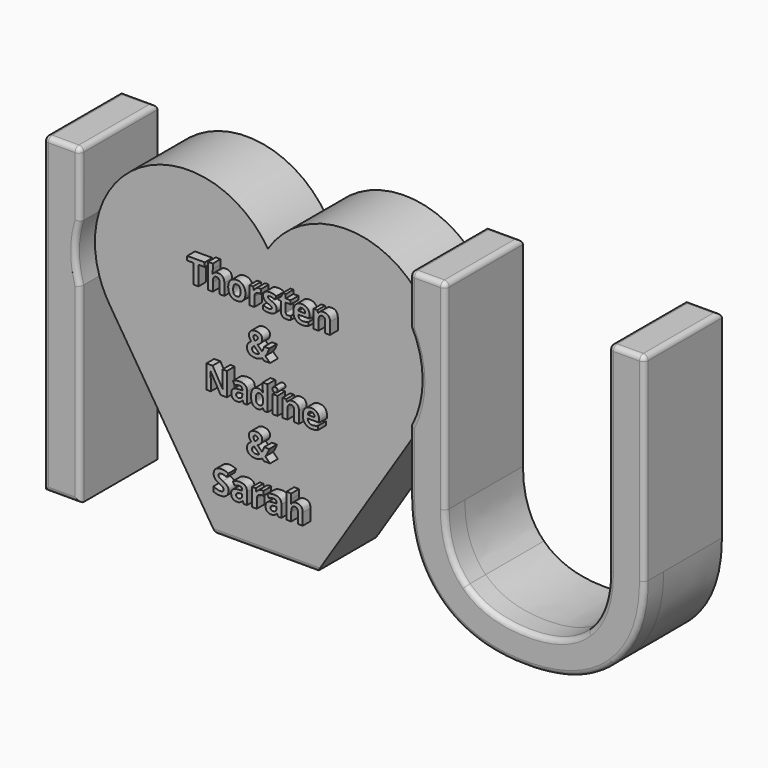
from build123d import *

# Parameters (mm, degrees)
F1_DEPTH     = 15
F2_TEXT_SIZE = 6.6989986393
F3_DEPTH     = 17
F4_R         = 1
F5_DEPTH     = 20
F6_R         = 1


# Not quite as in the source:
# - a feature names something its author has since deleted; it is built from what else it names
# - Text() gives the source's letters only with a copy of the font that has no kerning and outlines rounded to 1/6400 em; it was checked with that copy


with BuildPart() as f1:
    # F0 (on Front) → F1 (new body)
    with BuildSketch(Plane.XZ):
        with BuildLine():
            Line((-32.6601865779, 34.9033940146), (-10.6569835838, 0.1944517979))
            Line((-10.6569835838, 0.1944517979), (10.1186365179, 0.1944517979))
            Line((10.1186365179, 0.1944517979), (32.3398134221, 34.9033940146))
            ThreePointArc((32.3398134221, 34.9033940146), (32.7910788138, 35.6446323114), (33.2083891795, 36.4055046561))
            Line((33.2083891795, 36.4055046561), (33.2083891795, 54.1057090688))
            ThreePointArc((33.2083891795, 54.1057090688), (17.0374838295, 64.4358441872), (0, 55.6078197103))
            ThreePointArc((0, 55.6078197103), (-18.8035868283, 64.4316879893), (-34.7526041667, 51.1251341547))
            Line((-34.7526041667, 51.1251341547), (-34.7526041667, 39.3860795702))
            ThreePointArc((-34.7526041667, 39.3860795702), (-33.8503527488, 37.0775407014), (-32.6601865779, 34.9033940146))
        make_face()
        with BuildLine():
            Line((-34.7526041667, 0), (-34.7526041667, 39.3860795702))
            ThreePointArc((-34.7526041667, 39.3860795702), (-35.6650424142, 45.2556068624), (-34.7526041667, 51.1251341547))
            Line((-34.7526041667, 51.1251341547), (-34.7526041667, 64.4498697917))
            Line((-34.7526041667, 64.4498697917), (-42.2428385417, 64.4498697917))
            Line((-42.2428385417, 64.4498697917), (-42.2428385417, 0))
            Line((-42.2428385417, 0), (-34.7526041667, 0))
        make_face()
        with BuildLine():
            ThreePointArc((-34.7526041667, 51.1251341547), (-35.6650424142, 45.2556068624), (-34.7526041667, 39.3860795702))
            Line((-34.7526041667, 39.3860795702), (-34.7526041667, 51.1251341547))
        make_face()
        with BuildLine():
            Line((33.2083891795, 54.1057090688), (33.2083891795, 36.4055046561))
            ThreePointArc((33.2083891795, 36.4055046561), (35.3697555097, 45.2556068624), (33.2083891795, 54.1057090688))
        make_face()
        with BuildLine():
            ThreePointArc((33.2083891795, 54.1057090688), (35.3697555097, 45.2556068624), (33.2083891795, 36.4055046561))
            Line((33.2083891795, 36.4055046561), (33.2083891795, 23.742953204))
            add(Edge.make_bspline(
                [(39.4529606271, 6.6274334554), (33.2083891795, 12.8581741801), (33.2083891795, 23.742953204)],
                knots=[0, 0, 0, 1, 1, 1], degree=2))
            add(Edge.make_bspline(
                [(57.1078785739, 0.3966927308), (45.6975320748, 0.3966927308), (39.4529606271, 6.6274334554)],
                knots=[0, 0, 0, 1, 1, 1], degree=2))
            add(Edge.make_bspline(
                [(75.0463263427, 6.5790259248), (68.5182250729, 0.3966927308), (57.1078785739, 0.3966927308)],
                knots=[0, 0, 0, 1, 1, 1], degree=2))
            add(Edge.make_bspline(
                [(81.5744276124, 23.5769845277), (81.5744276124, 12.7613591189), (75.0463263427, 6.5790259248)],
                knots=[0, 0, 0, 1, 1, 1], degree=2))
            Line((81.5744276124, 23.5769845277), (81.5744276124, 64.4606018019))
            Line((81.5744276124, 64.4606018019), (74.230313684, 64.4606018019))
            Line((74.230313684, 64.4606018019), (74.230313684, 23.3142007901))
            add(Edge.make_bspline(
                [(69.9082127373, 11.1016723554), (74.230313684, 15.3615350483), (74.230313684, 23.3142007901)],
                knots=[0, 0, 0, 1, 1, 1], degree=2))
            add(Edge.make_bspline(
                [(57.5919538799, 6.8418096624), (65.5861117907, 6.8418096624), (69.9082127373, 11.1016723554)],
                knots=[0, 0, 0, 1, 1, 1], degree=2))
            add(Edge.make_bspline(
                [(44.8884347776, 11.0809262708), (49.2105357242, 6.8418096624), (57.5919538799, 6.8418096624)],
                knots=[0, 0, 0, 1, 1, 1], degree=2))
            add(Edge.make_bspline(
                [(40.566333831, 23.2312164519), (40.566333831, 15.3200428793), (44.8884347776, 11.0809262708)],
                knots=[0, 0, 0, 1, 1, 1], degree=2))
            Line((40.566333831, 23.2312164519), (40.566333831, 64.4606018019))
            Line((40.566333831, 64.4606018019), (33.2083891795, 64.4606018019))
            Line((33.2083891795, 64.4606018019), (33.2083891795, 54.1057090688))
        make_face()
    extrude(amount=F1_DEPTH)

    # F2 (on Front) → F3 (join)
    with BuildSketch(Plane.XZ):
        with Locations((-15.1669165656, 45.46367671)):
            Text('Thorsten', F2_TEXT_SIZE, font='Open Sans', font_style=FontStyle.BOLD, text_align=(TextAlign.LEFT, TextAlign.BOTTOM))
        with Locations((-2.9820660719, 36.3530385606)):
            Text('&', F2_TEXT_SIZE, font='Open Sans', font_style=FontStyle.BOLD, text_align=(TextAlign.LEFT, TextAlign.BOTTOM))
        with Locations((-11.6855307103, 27.2424004112)):
            Text('Nadine', F2_TEXT_SIZE, font='Open Sans', font_style=FontStyle.BOLD, text_align=(TextAlign.LEFT, TextAlign.BOTTOM))
        with Locations((-2.9820660719, 18.1317622618)):
            Text('&', F2_TEXT_SIZE, font='Open Sans', font_style=FontStyle.BOLD, text_align=(TextAlign.LEFT, TextAlign.BOTTOM))
        with Locations((-9.9448377826, 9.0211241124)):
            Text('Sarah', F2_TEXT_SIZE, font='Open Sans', font_style=FontStyle.BOLD, text_align=(TextAlign.LEFT, TextAlign.BOTTOM))
    extrude(amount=F3_DEPTH)

    # F4
    f4_edges = [f1.edges().sort_by_distance(p)[0] for p in [
        (-34.752604, -7.5, 64.44987),
        (-42.242839, -7.5, 64.44987),
        (-42.242839, -7.5, 0),
        (-34.752604, -7.5, 0),
        (-38.497721, 0, 64.44987),
        (-38.497721, 0, 0),
    ]]
    fillet(f4_edges, radius=F4_R)

    # F0 (on Front) → F5 (join)
    with BuildSketch(Plane.XZ):
        with BuildLine():
            Line((-34.7526041667, 0), (-34.7526041667, 39.3860795702))
            ThreePointArc((-34.7526041667, 39.3860795702), (-35.6650424142, 45.2556068624), (-34.7526041667, 51.1251341547))
            Line((-34.7526041667, 51.1251341547), (-34.7526041667, 64.4498697917))
            Line((-34.7526041667, 64.4498697917), (-42.2428385417, 64.4498697917))
            Line((-42.2428385417, 64.4498697917), (-42.2428385417, 0))
            Line((-42.2428385417, 0), (-34.7526041667, 0))
        make_face()
        with BuildLine():
            ThreePointArc((33.2083891795, 54.1057090688), (35.3697555097, 45.2556068624), (33.2083891795, 36.4055046561))
            Line((33.2083891795, 36.4055046561), (33.2083891795, 23.742953204))
            add(Edge.make_bspline(
                [(39.4529606271, 6.6274334554), (33.2083891795, 12.8581741801), (33.2083891795, 23.742953204)],
                knots=[0, 0, 0, 1, 1, 1], degree=2))
            add(Edge.make_bspline(
                [(57.1078785739, 0.3966927308), (45.6975320748, 0.3966927308), (39.4529606271, 6.6274334554)],
                knots=[0, 0, 0, 1, 1, 1], degree=2))
            add(Edge.make_bspline(
                [(75.0463263427, 6.5790259248), (68.5182250729, 0.3966927308), (57.1078785739, 0.3966927308)],
                knots=[0, 0, 0, 1, 1, 1], degree=2))
            add(Edge.make_bspline(
                [(81.5744276124, 23.5769845277), (81.5744276124, 12.7613591189), (75.0463263427, 6.5790259248)],
                knots=[0, 0, 0, 1, 1, 1], degree=2))
            Line((81.5744276124, 23.5769845277), (81.5744276124, 64.4606018019))
            Line((81.5744276124, 64.4606018019), (74.230313684, 64.4606018019))
            Line((74.230313684, 64.4606018019), (74.230313684, 23.3142007901))
            add(Edge.make_bspline(
                [(69.9082127373, 11.1016723554), (74.230313684, 15.3615350483), (74.230313684, 23.3142007901)],
                knots=[0, 0, 0, 1, 1, 1], degree=2))
            add(Edge.make_bspline(
                [(57.5919538799, 6.8418096624), (65.5861117907, 6.8418096624), (69.9082127373, 11.1016723554)],
                knots=[0, 0, 0, 1, 1, 1], degree=2))
            add(Edge.make_bspline(
                [(44.8884347776, 11.0809262708), (49.2105357242, 6.8418096624), (57.5919538799, 6.8418096624)],
                knots=[0, 0, 0, 1, 1, 1], degree=2))
            add(Edge.make_bspline(
                [(40.566333831, 23.2312164519), (40.566333831, 15.3200428793), (44.8884347776, 11.0809262708)],
                knots=[0, 0, 0, 1, 1, 1], degree=2))
            Line((40.566333831, 23.2312164519), (40.566333831, 64.4606018019))
            Line((40.566333831, 64.4606018019), (33.2083891795, 64.4606018019))
            Line((33.2083891795, 64.4606018019), (33.2083891795, 54.1057090688))
        make_face()
    extrude(amount=F5_DEPTH)

    # F6
    f6_edges = [f1.edges().sort_by_distance(p)[0] for p in [
        (-34.752604, -20, 19.69304),
        (-35.665042, -20, 45.255607),
        (-34.752604, -20, 57.787502),
        (-38.497721, -20, 64.44987),
        (-42.242839, -20, 32.224935),
        (-38.497721, -20, 0),
        (35.369756, -20, 45.255607),
        (33.208389, -20, 30.074229),
        (57.233936, -20, 0.396882),
        (81.574428, -20, 44.018793),
        (77.902371, -20, 64.460602),
        (74.230314, -20, 43.887401),
        (57.439259, -20, 6.842163),
        (40.566334, -20, 43.845909),
        (36.887362, -20, 64.460602),
        (33.208389, -20, 59.283155),
        (-10.656984, -7.5, 0.194452),
        (10.118637, -7.5, 0.194452),
        (-0.269174, 0, 0.194452),
        (-0.269174, -15, 0.194452),
        (81.574428, -10, 64.460602),
        (74.230314, -10, 64.460602),
        (77.902371, 0, 64.460602),
        (40.566334, -10, 64.460602),
        (33.208389, -10, 64.460602),
        (36.887362, 0, 64.460602),
        (-34.752604, -10, 64.44987),
        (-42.242839, -10, 64.44987),
        (-38.497721, 0, 64.44987),
    ]]
    fillet(f6_edges, radius=F6_R)


solid = f1.part
